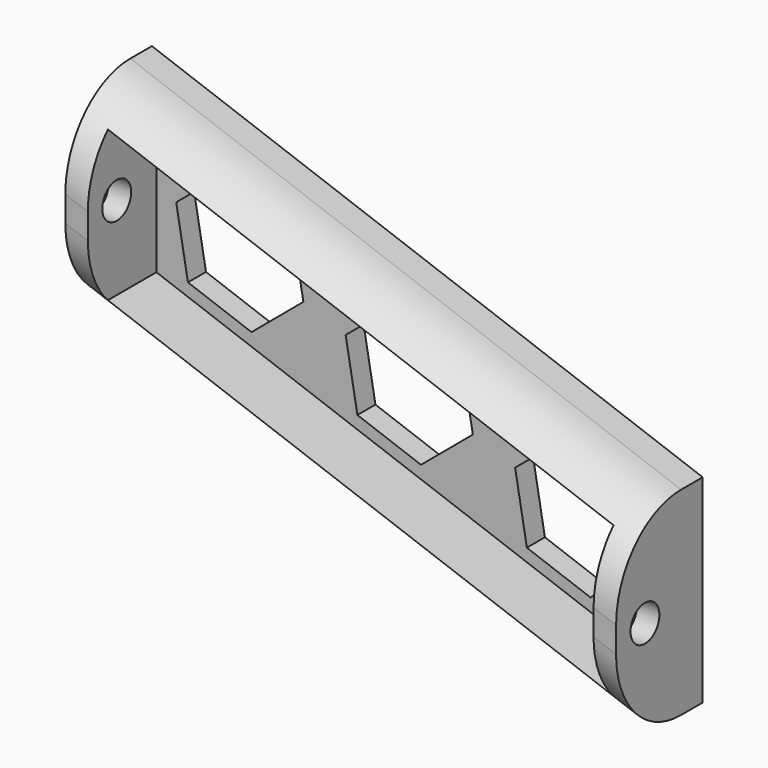
from build123d import *

# Parameters (mm, degrees)
F1_DEPTH    = 12
F2_T        = -2.5
F4_D        = 4
F4_DEPTH    = 6
F4_TIP      = 1.2017212381
F6_D        = 4
F6_DEPTH    = 6
F6_TIP      = 1.2017212381
F7_T1_DEPTH = 110
F7_T3_DEPTH = 110
F9_DEPTH    = 25


# Not quite as in the source:
# - a fillet or chamfer that OpenCascade refuses, or shapes differently, is made with other operations: its cross-section is extruded or revolved along the edge and cut away or added


with BuildPart() as f1:
    # F0 (on Front) → F1 (new body)
    with BuildSketch(Plane.XZ):
        Polygon((39.4877206884, 0), (-21.5922996627, 22.2313093162), (-21.5922996627, 0.2313093162), (39.4877206884, -22), align=None)
    extrude(amount=F1_DEPTH)

    # F2
    f2_openings = [f1.faces().sort_by_distance(p)[0] for p in [
        (8.947711, -12, 0.115655),
    ]]
    offset(amount=F2_T, openings=f2_openings)

    # F4
    with Locations(Plane(origin=(-21.5922996627, 0, 0), x_dir=(0, -1, 0), z_dir=(-1, 0, 0))):
        with Locations((8, 11.2313093162)):
            Hole(F4_D / 2, depth=F4_DEPTH)
            with Locations((0, 0, -(F4_DEPTH + F4_TIP / 2))):  # 118° drill point
                Cone(0, F4_D / 2, F4_TIP, mode=Mode.SUBTRACT)

    # F6
    with Locations(Plane.YZ.offset(39.4877206884)):
        with Locations((-8, -11)):
            Hole(F6_D / 2, depth=F6_DEPTH)
            with Locations((0, 0, -(F6_DEPTH + F6_TIP / 2))):  # 118° drill point
                Cone(0, F6_D / 2, F6_TIP, mode=Mode.SUBTRACT)

    # F7: fillet of radius 9 on 2 edges, made by hand

    # F7_s2 → F7_t1 (cut)
    with BuildSketch(Plane(origin=(56.0116188142, 0, -20.3865620214), x_dir=(0, 1, 0), z_dir=(-0.9396926208, 0, 0.3420201433))):
        with BuildLine():
            ThreePointArc((-3, -13.5055958894), (-9.3639610307, -10.8695569201), (-12, -4.5055958894))
            Line((-12, -4.5055958894), (-12, -13.5055958894))
            Line((-12, -13.5055958894), (-3, -13.5055958894))
        make_face()
    extrude(amount=F7_T1_DEPTH, mode=Mode.SUBTRACT)

    # F7_s4 → F7_t3 (cut)
    with BuildSketch(Plane(origin=(-40.2839057657, 0, 14.6621426187), x_dir=(0, 1, 0), z_dir=(0.9396926208, 0, -0.3420201433))):
        with BuildLine():
            ThreePointArc((-12, 1.8323582321), (-9.3639610307, -4.5316027985), (-3, -7.1676417679))
            Line((-3, -7.1676417679), (-12, -7.1676417679))
            Line((-12, -7.1676417679), (-12, 1.8323582321))
        make_face()
    extrude(amount=F7_T3_DEPTH, mode=Mode.SUBTRACT)

    # F8 (on face) → F9 (cut)
    with BuildSketch(Plane.XZ.offset(2.5)):
        Polygon((-8.5428162153, -0.4354697523), (-2.7932286645, 4.389007041), (-4.0965543521, 11.7805343179), (-11.1494675905, 14.3475848015), (-16.8990551413, 9.5231080082), (-15.5957294537, 2.1315807313), align=None)
        Polygon((10.2510362004, -7.2758726188), (16.0006237512, -2.4513958255), (14.6972980636, 4.9401314514), (7.6443848253, 7.507181935), (1.8947972745, 2.6827051417), (3.198122962, -4.7088221352), align=None)
        Polygon((29.0448886161, -14.1162754854), (34.7944761669, -9.2917986921), (33.4911504793, -1.9002714151), (26.438237241, 0.6667790685), (20.6886496902, -4.1576977248), (21.9919753777, -11.5492250017), align=None)
    extrude(amount=-F9_DEPTH, mode=Mode.SUBTRACT)


solid = f1.part
